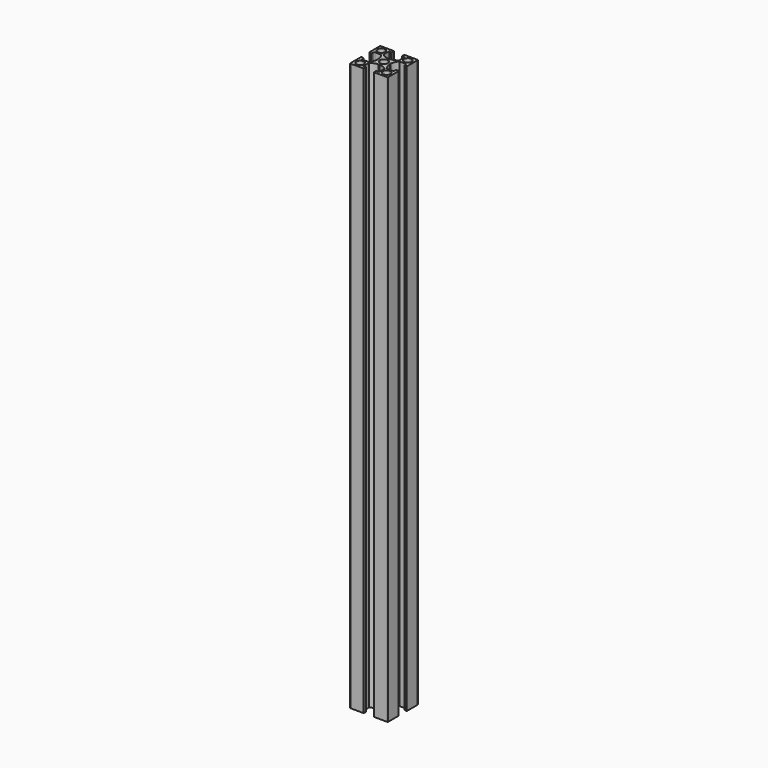
from build123d import *

# Parameters (mm, degrees)
F1_DEPTH = 300


# Not quite as in the source:
# - ends of sketch curves that miss each other by under 0.0002 mm in the source are joined


with BuildPart() as f1:
    # F0 (on Top) → F1 (new body)
    with BuildSketch(Plane.XY):
        with BuildLine():
            ThreePointArc((-2.15, 0), (-1.5202795796, 1.5202795796), (0, 2.15))
            Line((0, 2.15), (0, 3))
            Line((0, 3), (-0.307277, 3.307278))
            ThreePointArc((-0.307277, 3.307278), (-2.2820211583, 3.7143800615), (-4.036565823, 4.7078182229))
            ThreePointArc((-4.036565823, 4.7078182229), (-4.1201572004, 4.8123081084), (-4.15, 4.94275))
            Line((-4.15, 4.94275), (-4.15, 8.2))
            ThreePointArc((-4.15, 8.2), (-4.0621320344, 8.4121320344), (-3.85, 8.5))
            Line((-3.85, 8.5), (-2.95, 8.5))
            ThreePointArc((-2.95, 8.5), (-2.7378679656, 8.5878679656), (-2.65, 8.8))
            Line((-2.65, 8.8), (-2.65, 9.7))
            ThreePointArc((-2.65, 9.7), (-2.7378679656, 9.9121320344), (-2.95, 10))
            Line((-2.95, 10), (-9.7, 10))
            ThreePointArc((-9.7, 10), (-9.9121320344, 9.9121320344), (-10, 9.7))
            Line((-10, 9.7), (-10, 2.95))
            ThreePointArc((-10, 2.95), (-9.9121320344, 2.7378679656), (-9.7, 2.65))
            Line((-9.7, 2.65), (-8.8, 2.65))
            ThreePointArc((-8.8, 2.65), (-8.5878679656, 2.7378679656), (-8.5, 2.95))
            Line((-8.5, 2.95), (-8.5, 3.85))
            ThreePointArc((-8.5, 3.85), (-8.4121320344, 4.0621320344), (-8.2, 4.15))
            Line((-8.2, 4.15), (-4.942749, 4.15))
            ThreePointArc((-4.942749, 4.15), (-4.812307461, 4.1201573706), (-4.7078173786, 4.0365666993))
            ThreePointArc((-4.7078173786, 4.0365666993), (-3.7143793747, 2.2820219924), (-3.3072773955, 0.3072779813))
            Line((-3.3072773955, 0.3072779813), (-3, 0))
            Line((-3, 0), (-2.15, 0))
        make_face()
        with BuildLine():
            ThreePointArc((-7, 5), (-8.4142135624, 5.5857864376), (-9, 7))
            ThreePointArc((-9, 7), (-8.4142135624, 8.4142135624), (-7, 9))
            ThreePointArc((-7, 9), (-5.5857864376, 8.4142135624), (-5, 7))
            ThreePointArc((-5, 7), (-5.5857864376, 5.5857864376), (-7, 5))
        make_face(mode=Mode.SUBTRACT)
        with BuildLine():
            ThreePointArc((0, 2.15), (1.5202795796, 1.5202795796), (2.15, 0))
            Line((2.15, 0), (3, 0))
            Line((3, 0), (3.307278, 0.307278))
            ThreePointArc((3.307278, 0.307278), (3.7143803747, 2.2820219924), (4.7078187099, 4.0365664363))
            ThreePointArc((4.7078187099, 4.0365664363), (4.812308461, 4.1201573706), (4.94275, 4.15))
            Line((4.94275, 4.15), (8.2, 4.15))
            ThreePointArc((8.2, 4.15), (8.4121320344, 4.0621320344), (8.5, 3.85))
            Line((8.5, 3.85), (8.5, 2.95))
            ThreePointArc((8.5, 2.95), (8.5878679656, 2.7378679656), (8.8, 2.65))
            Line((8.8, 2.65), (9.7, 2.65))
            ThreePointArc((9.7, 2.65), (9.9121320344, 2.7378679656), (10, 2.95))
            Line((10, 2.95), (10, 9.7))
            ThreePointArc((10, 9.7), (9.9121320344, 9.9121320344), (9.7, 10))
            Line((9.7, 10), (2.95, 10))
            ThreePointArc((2.95, 10), (2.7378679656, 9.9121320344), (2.65, 9.7))
            Line((2.65, 9.7), (2.65, 8.8))
            ThreePointArc((2.65, 8.8), (2.7378679656, 8.5878679656), (2.95, 8.5))
            Line((2.95, 8.5), (3.85, 8.5))
            ThreePointArc((3.85, 8.5), (4.0621320344, 8.4121320344), (4.15, 8.2))
            Line((4.15, 8.2), (4.15, 4.94275))
            ThreePointArc((4.15, 4.94275), (4.1201572004, 4.8123081084), (4.036566086, 4.7078178916))
            ThreePointArc((4.036566086, 4.7078178916), (2.2820216259, 3.7143802371), (0.3072779813, 3.3072783955))
            Line((0.3072779813, 3.3072783955), (0, 3))
            Line((0, 3), (0, 2.15))
        make_face()
        with BuildLine():
            ThreePointArc((7, 9), (8.4142135624, 8.4142135624), (9, 7))
            ThreePointArc((9, 7), (8.4142135624, 5.5857864376), (7, 5))
            ThreePointArc((7, 5), (5.5857864376, 5.5857864376), (5, 7))
            ThreePointArc((5, 7), (5.5857864376, 8.4142135624), (7, 9))
        make_face(mode=Mode.SUBTRACT)
        with BuildLine():
            Line((3, 0), (2.15, 0))
            ThreePointArc((2.15, 0), (1.5202795796, -1.5202795796), (0, -2.15))
            Line((0, -2.15), (0, -3))
            Line((0, -3), (0.307278, -3.307277))
            ThreePointArc((0.307278, -3.307277), (2.2820216259, -3.7143792371), (4.036565823, -4.7078172229))
            ThreePointArc((4.036565823, -4.7078172229), (4.1201572004, -4.8123071084), (4.15, -4.942749))
            Line((4.15, -4.942749), (4.15, -8.2))
            ThreePointArc((4.15, -8.2), (4.0621320344, -8.4121320344), (3.85, -8.5))
            Line((3.85, -8.5), (2.95, -8.5))
            ThreePointArc((2.95, -8.5), (2.7378679656, -8.5878679656), (2.65, -8.8))
            Line((2.65, -8.8), (2.65, -9.7))
            ThreePointArc((2.65, -9.7), (2.7378679656, -9.9121320344), (2.95, -10))
            Line((2.95, -10), (9.7, -10))
            ThreePointArc((9.7, -10), (9.9121320344, -9.9121320344), (10, -9.7))
            Line((10, -9.7), (10, -2.95))
            ThreePointArc((10, -2.95), (9.9121320344, -2.7378679656), (9.7, -2.65))
            Line((9.7, -2.65), (8.8, -2.65))
            ThreePointArc((8.8, -2.65), (8.5878679656, -2.7378679656), (8.5, -2.95))
            Line((8.5, -2.95), (8.5, -3.85))
            ThreePointArc((8.5, -3.85), (8.4121320344, -4.0621320344), (8.2, -4.15))
            Line((8.2, -4.15), (4.94275, -4.15))
            ThreePointArc((4.94275, -4.15), (4.8123081084, -4.1201572004), (4.7078178916, -4.036566086))
            ThreePointArc((4.7078178916, -4.036566086), (3.7143800615, -2.2820211583), (3.3072783483, -0.3072769835))
            Line((3.3072783483, -0.3072769835), (3, 0))
        make_face()
        with BuildLine():
            ThreePointArc((7, -5), (8.4142135624, -5.5857864376), (9, -7))
            ThreePointArc((9, -7), (8.4142135624, -8.4142135624), (7, -9))
            ThreePointArc((7, -9), (5.5857864376, -8.4142135624), (5, -7))
            ThreePointArc((5, -7), (5.5857864376, -5.5857864376), (7, -5))
        make_face(mode=Mode.SUBTRACT)
        with BuildLine():
            Line((0, -3), (0, -2.15))
            ThreePointArc((0, -2.15), (-1.5202795796, -1.5202795796), (-2.15, 0))
            Line((-2.15, 0), (-3, 0))
            Line((-3, 0), (-3.307277, -0.307277))
            ThreePointArc((-3.307277, -0.307277), (-3.7143790615, -2.2820211583), (-4.7078172229, -4.036565823))
            ThreePointArc((-4.7078172229, -4.036565823), (-4.8123071084, -4.1201572004), (-4.942749, -4.15))
            Line((-4.942749, -4.15), (-8.2, -4.15))
            ThreePointArc((-8.2, -4.15), (-8.4121320344, -4.0621320344), (-8.5, -3.85))
            Line((-8.5, -3.85), (-8.5, -2.95))
            ThreePointArc((-8.5, -2.95), (-8.5878679656, -2.7378679656), (-8.8, -2.65))
            Line((-8.8, -2.65), (-9.7, -2.65))
            ThreePointArc((-9.7, -2.65), (-9.9121320344, -2.7378679656), (-10, -2.95))
            Line((-10, -2.95), (-10, -9.7))
            ThreePointArc((-10, -9.7), (-9.9121320344, -9.9121320344), (-9.7, -10))
            Line((-9.7, -10), (-2.95, -10))
            ThreePointArc((-2.95, -10), (-2.7378679656, -9.9121320344), (-2.65, -9.7))
            Line((-2.65, -9.7), (-2.65, -8.8))
            ThreePointArc((-2.65, -8.8), (-2.7378679656, -8.5878679656), (-2.95, -8.5))
            Line((-2.95, -8.5), (-3.85, -8.5))
            ThreePointArc((-3.85, -8.5), (-4.0621320344, -8.4121320344), (-4.15, -8.2))
            Line((-4.15, -8.2), (-4.15, -4.942749))
            ThreePointArc((-4.15, -4.942749), (-4.1201572004, -4.8123071084), (-4.036566086, -4.7078168916))
            ThreePointArc((-4.036566086, -4.7078168916), (-2.2820211583, -3.7143790615), (-0.3072769835, -3.3072773483))
            Line((-0.3072769835, -3.3072773483), (0, -3))
        make_face()
        with BuildLine():
            ThreePointArc((-7, -9), (-8.4142135624, -8.4142135624), (-9, -7))
            ThreePointArc((-9, -7), (-8.4142135624, -5.5857864376), (-7, -5))
            ThreePointArc((-7, -5), (-5.5857864376, -5.5857864376), (-5, -7))
            ThreePointArc((-5, -7), (-5.5857864376, -8.4142135624), (-7, -9))
        make_face(mode=Mode.SUBTRACT)
    extrude(amount=F1_DEPTH)


solid = f1.part
